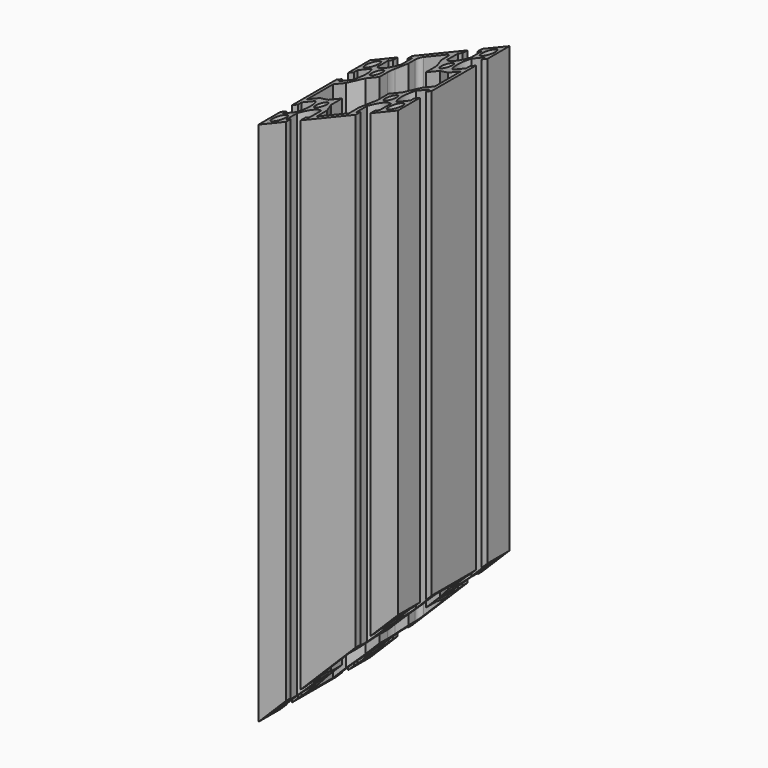
from build123d import *

# Parameters (mm, degrees)
F0_R          = 3
F0_R_2        = 2.5
F1_DEPTH      = 251
F2_R          = 2
F3_R          = 7
F6_DEPTH      = 30
F6_DEPTH_BACK = 30


# Not quite as in the source:
# - a feature names something its author has since deleted; it is built from what else it names


with BuildPart() as f1:
    # F0 (on Top) → F1 (new body)
    with BuildSketch(Plane.XY):
        with BuildLine():
            Line((18.15, -30), (30, -30))
            Line((30, -30), (30, -18.15))
            Line((30, -18.15), (27.5, -18.15))
            Line((27.5, -18.15), (27.5, -20.15))
            Line((27.5, -20.15), (21.5477069044, -20.15))
            ThreePointArc((21.5477069044, -20.15), (19.5, -15), (21.5477069044, -9.85))
            Line((21.5477069044, -9.85), (27.5, -9.85))
            Line((27.5, -9.85), (27.5, -11.85))
            Line((27.5, -11.85), (30, -11.85))
            Line((30, -11.85), (30, 11.85))
            Line((30, 11.85), (27.5, 11.85))
            Line((27.5, 11.85), (27.5, 9.85))
            Line((27.5, 9.85), (21.5477069044, 9.85))
            ThreePointArc((21.5477069044, 9.85), (19.5, 15), (21.5477069044, 20.15))
            Line((21.5477069044, 20.15), (27.5, 20.15))
            Line((27.5, 20.15), (27.5, 18.15))
            Line((27.5, 18.15), (30, 18.15))
            Line((30, 18.15), (30, 30))
            Line((30, 30), (18.15, 30))
            Line((18.15, 30), (18.15, 27.5))
            Line((18.15, 27.5), (20.15, 27.5))
            Line((20.15, 27.5), (20.15, 21.5477069044))
            ThreePointArc((20.15, 21.5477069044), (15, 19.5), (9.85, 21.5477069044))
            Line((9.85, 21.5477069044), (9.85, 27.5))
            Line((9.85, 27.5), (11.85, 27.5))
            Line((11.85, 27.5), (11.85, 30))
            Line((11.85, 30), (-11.85, 30))
            Line((-11.85, 30), (-11.85, 27.5))
            Line((-11.85, 27.5), (-9.85, 27.5))
            Line((-9.85, 27.5), (-9.85, 21.5477069044))
            ThreePointArc((-9.85, 21.5477069044), (-15, 19.5), (-20.15, 21.5477069044))
            Line((-20.15, 21.5477069044), (-20.15, 27.5))
            Line((-20.15, 27.5), (-18.15, 27.5))
            Line((-18.15, 27.5), (-18.15, 30))
            Line((-18.15, 30), (-30, 30))
            Line((-30, 30), (-30, 18.15))
            Line((-30, 18.15), (-27.5, 18.15))
            Line((-27.5, 18.15), (-27.5, 20.15))
            Line((-27.5, 20.15), (-21.5477069044, 20.15))
            ThreePointArc((-21.5477069044, 20.15), (-19.5, 15), (-21.5477069044, 9.85))
            Line((-21.5477069044, 9.85), (-27.5, 9.85))
            Line((-27.5, 9.85), (-27.5, 11.85))
            Line((-27.5, 11.85), (-30, 11.85))
            Line((-30, 11.85), (-30, -11.85))
            Line((-30, -11.85), (-27.5, -11.85))
            Line((-27.5, -11.85), (-27.5, -9.85))
            Line((-27.5, -9.85), (-21.5477069044, -9.85))
            ThreePointArc((-21.5477069044, -9.85), (-19.5, -15), (-21.5477069044, -20.15))
            Line((-21.5477069044, -20.15), (-27.5, -20.15))
            Line((-27.5, -20.15), (-27.5, -18.15))
            Line((-27.5, -18.15), (-30, -18.15))
            Line((-30, -18.15), (-30, -30))
            Line((-30, -30), (-18.15, -30))
            Line((-18.15, -30), (-18.15, -27.5))
            Line((-18.15, -27.5), (-20.15, -27.5))
            Line((-20.15, -27.5), (-20.15, -21.5477069044))
            ThreePointArc((-20.15, -21.5477069044), (-15, -19.5), (-9.85, -21.5477069044))
            Line((-9.85, -21.5477069044), (-9.85, -27.5))
            Line((-9.85, -27.5), (-11.85, -27.5))
            Line((-11.85, -27.5), (-11.85, -30))
            Line((-11.85, -30), (11.85, -30))
            Line((11.85, -30), (11.85, -27.5))
            Line((11.85, -27.5), (9.85, -27.5))
            Line((9.85, -27.5), (9.85, -21.5477069044))
            ThreePointArc((9.85, -21.5477069044), (15, -19.5), (20.15, -21.5477069044))
            Line((20.15, -21.5477069044), (20.15, -27.5))
            Line((20.15, -27.5), (18.15, -27.5))
            Line((18.15, -27.5), (18.15, -30))
        make_face()
        with Locations((-25, -25)):
            Circle(F0_R, mode=Mode.SUBTRACT)
        with Locations((-15, -15)):
            Circle(F0_R_2, mode=Mode.SUBTRACT)
        with Locations((25, -25)):
            Circle(F0_R, mode=Mode.SUBTRACT)
        with Locations((15, -15)):
            Circle(F0_R_2, mode=Mode.SUBTRACT)
        with Locations((-25, 25)):
            Circle(F0_R, mode=Mode.SUBTRACT)
        with Locations((-15, 15)):
            Circle(F0_R_2, mode=Mode.SUBTRACT)
        Polygon((-7, 22), (-7, 27.5), (0, 27.5), (7, 27.5), (7, 22), (10, 16), (10, 10), (16, 10), (22, 7), (27.5, 7), (27.5, 0), (27.5, -7), (22, -7), (16, -10), (10, -10), (10, -16), (7, -22), (7, -27.5), (0, -27.5), (-7, -27.5), (-7, -22), (-10, -16), (-10, -10), (-16, -10), (-22, -7), (-27.5, -7), (-27.5, 0), (-27.5, 7), (-22, 7), (-16, 10), (-10, 10), (-10, 16), align=None, mode=Mode.SUBTRACT)
        with Locations((15, 15)):
            Circle(F0_R_2, mode=Mode.SUBTRACT)
        with Locations((25, 25)):
            Circle(F0_R, mode=Mode.SUBTRACT)
    extrude(amount=F1_DEPTH)

    # F2
    f2_edges = [f1.edges().sort_by_distance(p)[0] for p in [
        (-7, 27.5, 125.5),
        (7, 27.5, 125.5),
    ]]
    fillet(f2_edges, radius=F2_R)

    # F3
    f3_edges = [f1.edges().sort_by_distance(p)[0] for p in [
        (-10, 16, 125.5),
        (10, 16, 125.5),
    ]]
    fillet(f3_edges, radius=F3_R)

    # F5 (on Front) → F6 (cut, two sides)
    with BuildSketch(Plane.XZ) as f6_sk:
        Polygon((-177.8936772938, 164.8876193333), (30, 251), (-52.9032198334, 451.1460776863), (-260.7968971272, 365.0336970195), align=None)
        Polygon((247.13668536, 46.6947819077), (131.9157336339, 161.9157336339), (-30, 0), (85.2209517261, -115.2209517261), align=None)
    extrude(amount=F6_DEPTH, mode=Mode.SUBTRACT)
    extrude(f6_sk.sketch, amount=-F6_DEPTH_BACK, mode=Mode.SUBTRACT)


solid = f1.part
